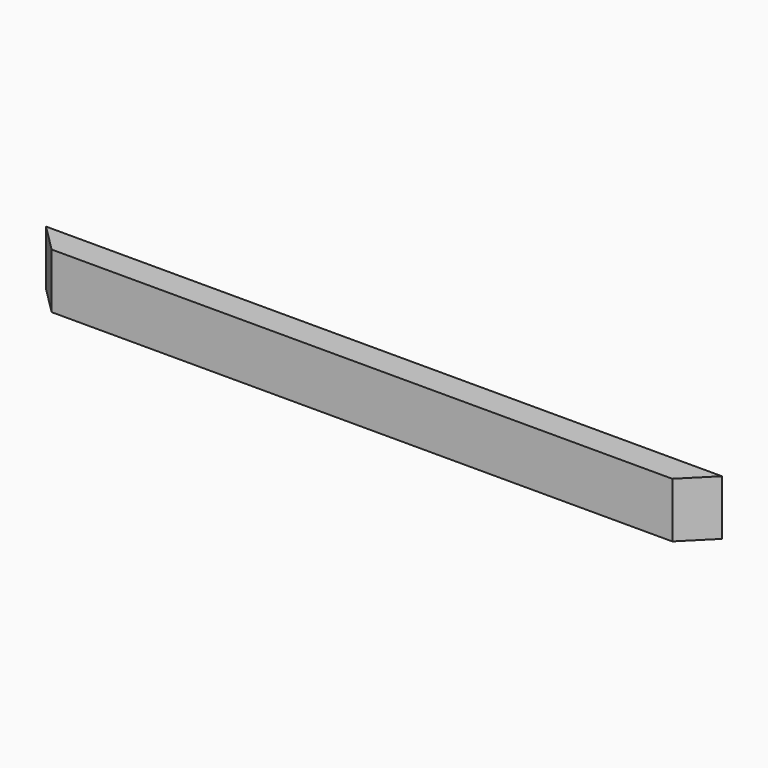
from build123d import *

# Parameters (mm, degrees)
F0_W     = 1244.6
F0_H     = 101.6
F3_DEPTH = 50.8
F1_SIZE  = 50.79999
F2_SIZE  = 50.79999


# Not quite as in the source:
# - a fillet or chamfer is up to 0.001 mm smaller than in the source, because OpenCascade refuses the exact size


with BuildPart() as f3:
    # F0 (on Front) → F3 (new body)
    with BuildSketch(Plane.XZ):
        with Locations((-28.0373948519, 50.8)):
            Rectangle(F0_W, F0_H)
    extrude(amount=F3_DEPTH)

    # F1 (size 50.8 in the source; OpenCascade refuses exactly that, so slightly less here)
    f1_edges = [f3.edges().sort_by_distance(p)[0] for p in [
        (594.262605, -50.8, 50.8),
    ]]
    chamfer(f1_edges, length=F1_SIZE)

    # F2 (size 50.8 in the source; OpenCascade refuses exactly that, so slightly less here)
    f2_edges = [f3.edges().sort_by_distance(p)[0] for p in [
        (-650.337395, -50.8, 50.8),
    ]]
    chamfer(f2_edges, length=F2_SIZE)


solid = f3.part
